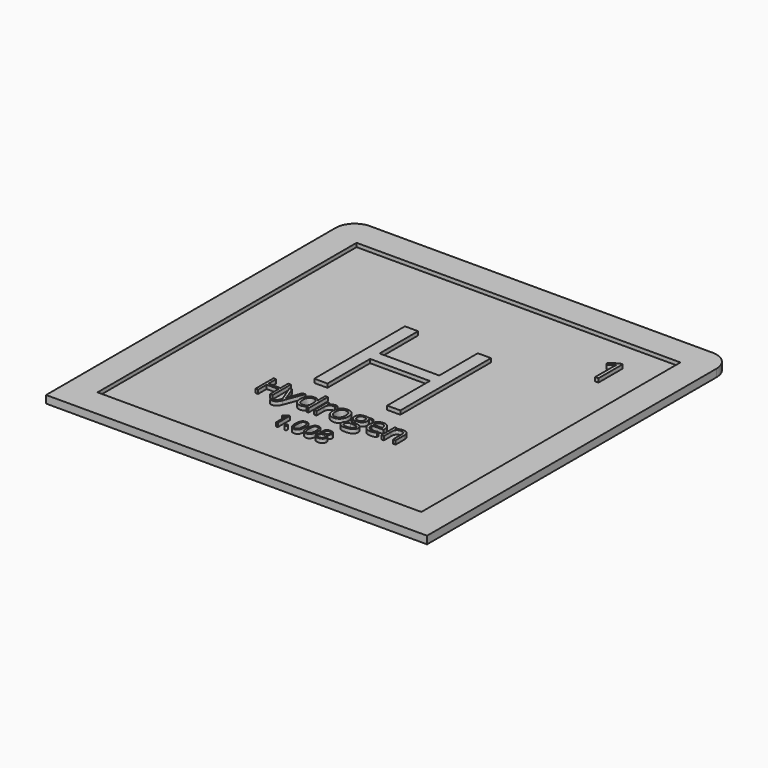
from build123d import *

# Parameters (mm, degrees)
F0_W           = 100
F0_H           = 100
F0_W_2         = 85
F0_H_2         = 85
F0_TEXT_SIZE   = 41.6666666667
F0_TEXT_SIZE_2 = 11.1111111111
F0_TEXT_SIZE_3 = 8.3333333333
F0_TEXT_SIZE_4 = 5.5555555556
F1_DEPTH       = 2
F2_R           = 5
F4_DEPTH       = 1


# Not quite as in the source:
# - Text() gives the source's letters only with a copy of the font that has no kerning and outlines rounded to 1/6400 em; it was checked with that copy


with BuildPart() as f1:
    # F0 (on Top) → F1 (new body)
    with BuildSketch(Plane.XY):
        Rectangle(F0_W, F0_H)
        Rectangle(F0_W_2, F0_H_2, mode=Mode.SUBTRACT)
        with Locations((-15.6875, -10)):
            Text('H', F0_TEXT_SIZE, font='Open Sans', text_align=(TextAlign.LEFT, TextAlign.BOTTOM))
        with Locations((29.9010416667, 26.5)):
            Text('1', F0_TEXT_SIZE_2, font='Open Sans', text_align=(TextAlign.LEFT, TextAlign.BOTTOM))
        with Locations((-19.0579427083, -21)):
            Text('Hydrogen', F0_TEXT_SIZE_3, font='Open Sans', text_align=(TextAlign.LEFT, TextAlign.BOTTOM))
        with Locations((-7.1280381944, -30)):
            Text('1.008', F0_TEXT_SIZE_4, font='Open Sans', text_align=(TextAlign.LEFT, TextAlign.BOTTOM))
    extrude(amount=F1_DEPTH)

    # F2
    f2_edges = [f1.edges().sort_by_distance(p)[0] for p in [
        (50, 50, 1),
        (-50, 50, 1),
    ]]
    fillet(f2_edges, radius=F2_R)

    # F0 (on Top) → F4 (join)
    with BuildSketch(Plane.XY):
        Rectangle(F0_W_2, F0_H_2)
        with BuildLine():
            add(Edge.make_bspline(
                [(-3.4487847222, -29.9934895833), (-3.5394965278, -29.9079861111), (-3.5394965278, -29.7126736111)],
                knots=[0, 0, 0, 1, 1, 1], degree=2))
            add(Edge.make_bspline(
                [(-3.5394965278, -29.7126736111), (-3.5394965278, -29.5303819444), (-3.4565972222, -29.4370659722)],
                knots=[0, 0, 0, 1, 1, 1], degree=2))
            add(Edge.make_bspline(
                [(-3.4565972222, -29.4370659722), (-3.3736979167, -29.34375), (-3.2191840278, -29.34375)],
                knots=[0, 0, 0, 1, 1, 1], degree=2))
            add(Edge.make_bspline(
                [(-3.2191840278, -29.34375), (-3.0620659722, -29.34375), (-2.9739583333, -29.4370659722)],
                knots=[0, 0, 0, 1, 1, 1], degree=2))
            add(Edge.make_bspline(
                [(-2.9739583333, -29.4370659722), (-2.8858506944, -29.5303819444), (-2.8858506944, -29.7126736111)],
                knots=[0, 0, 0, 1, 1, 1], degree=2))
            add(Edge.make_bspline(
                [(-2.8858506944, -29.7126736111), (-2.8858506944, -29.8888888889), (-2.9752604167, -29.9839409722)],
                knots=[0, 0, 0, 1, 1, 1], degree=2))
            add(Edge.make_bspline(
                [(-2.9752604167, -29.9839409722), (-3.0646701389, -30.0789930556), (-3.2191840278, -30.0789930556)],
                knots=[0, 0, 0, 1, 1, 1], degree=2))
            add(Edge.make_bspline(
                [(-3.2191840278, -30.0789930556), (-3.3580729167, -30.0789930556), (-3.4487847222, -29.9934895833)],
                knots=[0, 0, 0, 1, 1, 1], degree=2))
        make_face(mode=Mode.SUBTRACT)
        with BuildLine():
            Line((-5.1888020833, -26.0338541667), (-5.1888020833, -30))
            Line((-5.1888020833, -30), (-5.6280381944, -30))
            Line((-5.6280381944, -30), (-5.6280381944, -27.1736111111))
            add(Edge.make_bspline(
                [(-5.6280381944, -27.1736111111), (-5.6280381944, -26.8203125), (-5.6063368056, -26.5060763889)],
                knots=[0, 0, 0, 1, 1, 1], degree=2))
            add(Edge.make_bspline(
                [(-5.6063368056, -26.5060763889), (-5.6627604167, -26.5633680556), (-5.7335069444, -26.6254340278)],
                knots=[0, 0, 0, 1, 1, 1], degree=2))
            add(Edge.make_bspline(
                [(-5.7335069444, -26.6254340278), (-5.8042534722, -26.6875), (-6.37890625, -27.1545138889)],
                knots=[0, 0, 0, 1, 1, 1], degree=2))
            Line((-6.37890625, -27.1545138889), (-6.6176215278, -26.8454861111))
            Line((-6.6176215278, -26.8454861111), (-5.5681423611, -26.0338541667))
            Line((-5.5681423611, -26.0338541667), (-5.1888020833, -26.0338541667))
        make_face(mode=Mode.SUBTRACT)
        with BuildLine():
            add(Edge.make_bspline(
                [(0.0915798611, -26.4952256944), (0.4266493056, -27.0190972222), (0.4266493056, -28.0112847222)],
                knots=[0, 0, 0, 1, 1, 1], degree=2))
            add(Edge.make_bspline(
                [(0.4266493056, -28.0112847222), (0.4266493056, -29.0399305556), (0.1024305556, -29.5473090278)],
                knots=[0, 0, 0, 1, 1, 1], degree=2))
            add(Edge.make_bspline(
                [(0.1024305556, -29.5473090278), (-0.2217881944, -30.0546875), (-0.8893229167, -30.0546875)],
                knots=[0, 0, 0, 1, 1, 1], degree=2))
            add(Edge.make_bspline(
                [(-0.8893229167, -30.0546875), (-1.5290798611, -30.0546875), (-1.8628472222, -29.53515625)],
                knots=[0, 0, 0, 1, 1, 1], degree=2))
            add(Edge.make_bspline(
                [(-1.8628472222, -29.53515625), (-2.1966145833, -29.015625), (-2.1966145833, -28.0112847222)],
                knots=[0, 0, 0, 1, 1, 1], degree=2))
            add(Edge.make_bspline(
                [(-2.1966145833, -28.0112847222), (-2.1966145833, -26.9756944444), (-1.8736979167, -26.4735243056)],
                knots=[0, 0, 0, 1, 1, 1], degree=2))
            add(Edge.make_bspline(
                [(-1.8736979167, -26.4735243056), (-1.55078125, -25.9713541667), (-0.8893229167, -25.9713541667)],
                knots=[0, 0, 0, 1, 1, 1], degree=2))
            add(Edge.make_bspline(
                [(-0.8893229167, -25.9713541667), (-0.2434895833, -25.9713541667), (0.0915798611, -26.4952256944)],
                knots=[0, 0, 0, 1, 1, 1], degree=2))
        make_face(mode=Mode.SUBTRACT)
        Polygon((-13.7233072917, -15.05078125), (-13.7233072917, -21), (-14.4147135417, -21), (-14.4147135417, -18.2005208333), (-17.548828125, -18.2005208333), (-17.548828125, -21), (-18.240234375, -21), (-18.240234375, -15.05078125), (-17.548828125, -15.05078125), (-17.548828125, -17.58203125), (-14.4147135417, -17.58203125), (-14.4147135417, -15.05078125), align=None, mode=Mode.SUBTRACT)
        with BuildLine():
            Line((-11.1022135417, -21.0247395833), (-12.9016927083, -16.5403645833))
            Line((-12.9016927083, -16.5403645833), (-12.1764322917, -16.5403645833))
            Line((-12.1764322917, -16.5403645833), (-11.1998697917, -19.0833333333))
            add(Edge.make_bspline(
                [(-11.1998697917, -19.0833333333), (-10.8795572917, -19.9544270833), (-10.8014322917, -20.3411458333)],
                knots=[0, 0, 0, 1, 1, 1], degree=2))
            Line((-10.8014322917, -20.3411458333), (-10.7688802083, -20.3411458333))
            add(Edge.make_bspline(
                [(-10.7688802083, -20.3411458333), (-10.716796875, -20.1328125), (-10.5475260417, -19.6302083333)],
                knots=[0, 0, 0, 1, 1, 1], degree=2))
            add(Edge.make_bspline(
                [(-10.5475260417, -19.6302083333), (-10.3782552083, -19.1276041667), (-9.4420572917, -16.5403645833)],
                knots=[0, 0, 0, 1, 1, 1], degree=2))
            Line((-9.4420572917, -16.5403645833), (-8.7180989583, -16.5403645833))
            Line((-8.7180989583, -16.5403645833), (-10.634765625, -21.6184895833))
            add(Edge.make_bspline(
                [(-10.634765625, -21.6184895833), (-10.919921875, -22.37109375), (-11.3001302083, -22.6868489583)],
                knots=[0, 0, 0, 1, 1, 1], degree=2))
            add(Edge.make_bspline(
                [(-11.3001302083, -22.6868489583), (-11.6803385417, -23.0026041667), (-12.2337239583, -23.0026041667)],
                knots=[0, 0, 0, 1, 1, 1], degree=2))
            add(Edge.make_bspline(
                [(-12.2337239583, -23.0026041667), (-12.5436197917, -23.0026041667), (-12.8444010417, -22.9322916667)],
                knots=[0, 0, 0, 1, 1, 1], degree=2))
            Line((-12.8444010417, -22.9322916667), (-12.8444010417, -22.3919270833))
            add(Edge.make_bspline(
                [(-12.8444010417, -22.3919270833), (-12.6204427083, -22.4401041667), (-12.3444010417, -22.4401041667)],
                knots=[0, 0, 0, 1, 1, 1], degree=2))
            add(Edge.make_bspline(
                [(-12.3444010417, -22.4401041667), (-11.6477864583, -22.4401041667), (-11.3509114583, -21.6588541667)],
                knots=[0, 0, 0, 1, 1, 1], degree=2))
            Line((-11.3509114583, -21.6588541667), (-11.1022135417, -21.0247395833))
        make_face(mode=Mode.SUBTRACT)
        with BuildLine():
            Line((-4.869140625, -21), (-4.958984375, -20.40234375))
            Line((-4.958984375, -20.40234375), (-4.9954427083, -20.40234375))
            add(Edge.make_bspline(
                [(-4.9954427083, -20.40234375), (-5.462890625, -21.08203125), (-6.3951822917, -21.08203125)],
                knots=[0, 0, 0, 1, 1, 1], degree=2))
            add(Edge.make_bspline(
                [(-6.3951822917, -21.08203125), (-7.2701822917, -21.08203125), (-7.7565104167, -20.4837239583)],
                knots=[0, 0, 0, 1, 1, 1], degree=2))
            add(Edge.make_bspline(
                [(-7.7565104167, -20.4837239583), (-8.2428385417, -19.8854166667), (-8.2428385417, -18.7825520833)],
                knots=[0, 0, 0, 1, 1, 1], degree=2))
            add(Edge.make_bspline(
                [(-8.2428385417, -18.7825520833), (-8.2428385417, -17.6796875), (-7.7545572917, -17.0690104167)],
                knots=[0, 0, 0, 1, 1, 1], degree=2))
            add(Edge.make_bspline(
                [(-7.7545572917, -17.0690104167), (-7.2662760417, -16.4583333333), (-6.3951822917, -16.4583333333)],
                knots=[0, 0, 0, 1, 1, 1], degree=2))
            add(Edge.make_bspline(
                [(-6.3951822917, -16.4583333333), (-5.4876302083, -16.4583333333), (-5.0032552083, -17.1184895833)],
                knots=[0, 0, 0, 1, 1, 1], degree=2))
            Line((-5.0032552083, -17.1184895833), (-4.9498697917, -17.1184895833))
            Line((-4.9498697917, -17.1184895833), (-4.978515625, -16.796875))
            Line((-4.978515625, -16.796875), (-4.9954427083, -16.4830729167))
            Line((-4.9954427083, -16.4830729167), (-4.9954427083, -14.66796875))
            Line((-4.9954427083, -14.66796875), (-4.3196614583, -14.66796875))
            Line((-4.3196614583, -14.66796875), (-4.3196614583, -21))
            Line((-4.3196614583, -21), (-4.869140625, -21))
        make_face(mode=Mode.SUBTRACT)
        with BuildLine():
            add(Edge.make_bspline(
                [(-1.6217447917, -16.6946614583), (-1.271484375, -16.4583333333), (-0.8522135417, -16.4583333333)],
                knots=[0, 0, 0, 1, 1, 1], degree=2))
            add(Edge.make_bspline(
                [(-0.8522135417, -16.4583333333), (-0.5553385417, -16.4583333333), (-0.3196614583, -16.5078125)],
                knots=[0, 0, 0, 1, 1, 1], degree=2))
            Line((-0.3196614583, -16.5078125), (-0.4134114583, -17.1341145833))
            add(Edge.make_bspline(
                [(-0.4134114583, -17.1341145833), (-0.689453125, -17.0729166667), (-0.9016927083, -17.0729166667)],
                knots=[0, 0, 0, 1, 1, 1], degree=2))
            add(Edge.make_bspline(
                [(-0.9016927083, -17.0729166667), (-1.443359375, -17.0729166667), (-1.8274739583, -17.5123697917)],
                knots=[0, 0, 0, 1, 1, 1], degree=2))
            add(Edge.make_bspline(
                [(-1.8274739583, -17.5123697917), (-2.2115885417, -17.9518229167), (-2.2115885417, -18.6067708333)],
                knots=[0, 0, 0, 1, 1, 1], degree=2))
            Line((-2.2115885417, -18.6067708333), (-2.2115885417, -21))
            Line((-2.2115885417, -21), (-2.8873697917, -21))
            Line((-2.8873697917, -21), (-2.8873697917, -16.5403645833))
            Line((-2.8873697917, -16.5403645833), (-2.330078125, -16.5403645833))
            Line((-2.330078125, -16.5403645833), (-2.251953125, -17.3658854167))
            Line((-2.251953125, -17.3658854167), (-2.2194010417, -17.3658854167))
            add(Edge.make_bspline(
                [(-2.2194010417, -17.3658854167), (-1.9720052083, -16.9309895833), (-1.6217447917, -16.6946614583)],
                knots=[0, 0, 0, 1, 1, 1], degree=2))
        make_face(mode=Mode.SUBTRACT)
        with BuildLine():
            add(Edge.make_bspline(
                [(3.2677951389, -26.4952256944), (3.6028645833, -27.0190972222), (3.6028645833, -28.0112847222)],
                knots=[0, 0, 0, 1, 1, 1], degree=2))
            add(Edge.make_bspline(
                [(3.6028645833, -28.0112847222), (3.6028645833, -29.0399305556), (3.2786458333, -29.5473090278)],
                knots=[0, 0, 0, 1, 1, 1], degree=2))
            add(Edge.make_bspline(
                [(3.2786458333, -29.5473090278), (2.9544270833, -30.0546875), (2.2868923611, -30.0546875)],
                knots=[0, 0, 0, 1, 1, 1], degree=2))
            add(Edge.make_bspline(
                [(2.2868923611, -30.0546875), (1.6471354167, -30.0546875), (1.3133680556, -29.53515625)],
                knots=[0, 0, 0, 1, 1, 1], degree=2))
            add(Edge.make_bspline(
                [(1.3133680556, -29.53515625), (0.9796006944, -29.015625), (0.9796006944, -28.0112847222)],
                knots=[0, 0, 0, 1, 1, 1], degree=2))
            add(Edge.make_bspline(
                [(0.9796006944, -28.0112847222), (0.9796006944, -26.9756944444), (1.3025173611, -26.4735243056)],
                knots=[0, 0, 0, 1, 1, 1], degree=2))
            add(Edge.make_bspline(
                [(1.3025173611, -26.4735243056), (1.6254340278, -25.9713541667), (2.2868923611, -25.9713541667)],
                knots=[0, 0, 0, 1, 1, 1], degree=2))
            add(Edge.make_bspline(
                [(2.2868923611, -25.9713541667), (2.9327256944, -25.9713541667), (3.2677951389, -26.4952256944)],
                knots=[0, 0, 0, 1, 1, 1], degree=2))
        make_face(mode=Mode.SUBTRACT)
        with BuildLine():
            add(Edge.make_bspline(
                [(4.6098090278, -26.2335069444), (4.9283854167, -25.9774305556), (5.4631076389, -25.9774305556)],
                knots=[0, 0, 0, 1, 1, 1], degree=2))
            add(Edge.make_bspline(
                [(5.4631076389, -25.9774305556), (6.0056423611, -25.9774305556), (6.3229166667, -26.2296006944)],
                knots=[0, 0, 0, 1, 1, 1], degree=2))
            add(Edge.make_bspline(
                [(6.3229166667, -26.2296006944), (6.6401909722, -26.4817708333), (6.6401909722, -26.9262152778)],
                knots=[0, 0, 0, 1, 1, 1], degree=2))
            add(Edge.make_bspline(
                [(6.6401909722, -26.9262152778), (6.6401909722, -27.2196180556), (6.4587673611, -27.4609375)],
                knots=[0, 0, 0, 1, 1, 1], degree=2))
            add(Edge.make_bspline(
                [(6.4587673611, -27.4609375), (6.27734375, -27.7022569444), (5.8780381944, -27.9001736111)],
                knots=[0, 0, 0, 1, 1, 1], degree=2))
            add(Edge.make_bspline(
                [(5.8780381944, -27.9001736111), (6.3606770833, -28.1310763889), (6.5642361111, -28.3845486111)],
                knots=[0, 0, 0, 1, 1, 1], degree=2))
            add(Edge.make_bspline(
                [(6.5642361111, -28.3845486111), (6.7677951389, -28.6380208333), (6.7677951389, -28.9722222222)],
                knots=[0, 0, 0, 1, 1, 1], degree=2))
            add(Edge.make_bspline(
                [(6.7677951389, -28.9722222222), (6.7677951389, -29.4652777778), (6.4231770833, -29.7599826389)],
                knots=[0, 0, 0, 1, 1, 1], degree=2))
            add(Edge.make_bspline(
                [(6.4231770833, -29.7599826389), (6.0785590278, -30.0546875), (5.4796006944, -30.0546875)],
                knots=[0, 0, 0, 1, 1, 1], degree=2))
            add(Edge.make_bspline(
                [(5.4796006944, -30.0546875), (4.8450520833, -30.0546875), (4.5030381944, -29.7764756944)],
                knots=[0, 0, 0, 1, 1, 1], degree=2))
            add(Edge.make_bspline(
                [(4.5030381944, -29.7764756944), (4.1610243056, -29.4982638889), (4.1610243056, -28.9878472222)],
                knots=[0, 0, 0, 1, 1, 1], degree=2))
            add(Edge.make_bspline(
                [(4.1610243056, -28.9878472222), (4.1610243056, -28.3072916667), (4.9908854167, -27.9270833333)],
                knots=[0, 0, 0, 1, 1, 1], degree=2))
            add(Edge.make_bspline(
                [(4.9908854167, -27.9270833333), (4.6167534722, -27.7161458333), (4.4539930556, -27.4704861111)],
                knots=[0, 0, 0, 1, 1, 1], degree=2))
            add(Edge.make_bspline(
                [(4.4539930556, -27.4704861111), (4.2912326389, -27.2248263889), (4.2912326389, -26.9210069444)],
                knots=[0, 0, 0, 1, 1, 1], degree=2))
            add(Edge.make_bspline(
                [(4.2912326389, -26.9210069444), (4.2912326389, -26.4895833333), (4.6098090278, -26.2335069444)],
                knots=[0, 0, 0, 1, 1, 1], degree=2))
        make_face(mode=Mode.SUBTRACT)
        with BuildLine():
            add(Edge.make_bspline(
                [(3.8125, -17.0813802083), (4.3639322917, -17.7044270833), (4.3639322917, -18.765625)],
                knots=[0, 0, 0, 1, 1, 1], degree=2))
            add(Edge.make_bspline(
                [(4.3639322917, -18.765625), (4.3639322917, -19.8567708333), (3.8151041667, -20.4694010417)],
                knots=[0, 0, 0, 1, 1, 1], degree=2))
            add(Edge.make_bspline(
                [(3.8151041667, -20.4694010417), (3.2662760417, -21.08203125), (2.2975260417, -21.08203125)],
                knots=[0, 0, 0, 1, 1, 1], degree=2))
            add(Edge.make_bspline(
                [(2.2975260417, -21.08203125), (1.6985677083, -21.08203125), (1.2350260417, -20.80078125)],
                knots=[0, 0, 0, 1, 1, 1], degree=2))
            add(Edge.make_bspline(
                [(1.2350260417, -20.80078125), (0.771484375, -20.51953125), (0.5188802083, -19.9947916667)],
                knots=[0, 0, 0, 1, 1, 1], degree=2))
            add(Edge.make_bspline(
                [(0.5188802083, -19.9947916667), (0.2662760417, -19.4700520833), (0.2662760417, -18.765625)],
                knots=[0, 0, 0, 1, 1, 1], degree=2))
            add(Edge.make_bspline(
                [(0.2662760417, -18.765625), (0.2662760417, -17.67578125), (0.8118489583, -17.0670572917)],
                knots=[0, 0, 0, 1, 1, 1], degree=2))
            add(Edge.make_bspline(
                [(0.8118489583, -17.0670572917), (1.357421875, -16.4583333333), (2.326171875, -16.4583333333)],
                knots=[0, 0, 0, 1, 1, 1], degree=2))
            add(Edge.make_bspline(
                [(2.326171875, -16.4583333333), (3.2610677083, -16.4583333333), (3.8125, -17.0813802083)],
                knots=[0, 0, 0, 1, 1, 1], degree=2))
        make_face(mode=Mode.SUBTRACT)
        with BuildLine():
            Line((7.6569010417, -16.5403645833), (9.1985677083, -16.5403645833))
            Line((9.1985677083, -16.5403645833), (9.1985677083, -16.9674479167))
            Line((9.1985677083, -16.9674479167), (8.373046875, -17.0651041667))
            add(Edge.make_bspline(
                [(8.373046875, -17.0651041667), (8.486328125, -17.20703125), (8.576171875, -17.4375)],
                knots=[0, 0, 0, 1, 1, 1], degree=2))
            add(Edge.make_bspline(
                [(8.576171875, -17.4375), (8.666015625, -17.66796875), (8.666015625, -17.9557291667)],
                knots=[0, 0, 0, 1, 1, 1], degree=2))
            add(Edge.make_bspline(
                [(8.666015625, -17.9557291667), (8.666015625, -18.6119791667), (8.2180989583, -19.0026041667)],
                knots=[0, 0, 0, 1, 1, 1], degree=2))
            add(Edge.make_bspline(
                [(8.2180989583, -19.0026041667), (7.7701822917, -19.3932291667), (6.9889322917, -19.3932291667)],
                knots=[0, 0, 0, 1, 1, 1], degree=2))
            add(Edge.make_bspline(
                [(6.9889322917, -19.3932291667), (6.7897135417, -19.3932291667), (6.615234375, -19.3606770833)],
                knots=[0, 0, 0, 1, 1, 1], degree=2))
            add(Edge.make_bspline(
                [(6.615234375, -19.3606770833), (6.1842447917, -19.5885416667), (6.1842447917, -19.93359375)],
                knots=[0, 0, 0, 1, 1, 1], degree=2))
            add(Edge.make_bspline(
                [(6.1842447917, -19.93359375), (6.1842447917, -20.1171875), (6.3346354167, -20.2044270833)],
                knots=[0, 0, 0, 1, 1, 1], degree=2))
            add(Edge.make_bspline(
                [(6.3346354167, -20.2044270833), (6.4850260417, -20.2916666667), (6.8509114583, -20.2916666667)],
                knots=[0, 0, 0, 1, 1, 1], degree=2))
            Line((6.8509114583, -20.2916666667), (7.6399739583, -20.2916666667))
            add(Edge.make_bspline(
                [(7.6399739583, -20.2916666667), (8.365234375, -20.2916666667), (8.7532552083, -20.5970052083)],
                knots=[0, 0, 0, 1, 1, 1], degree=2))
            add(Edge.make_bspline(
                [(8.7532552083, -20.5970052083), (9.1412760417, -20.90234375), (9.1412760417, -21.484375)],
                knots=[0, 0, 0, 1, 1, 1], degree=2))
            add(Edge.make_bspline(
                [(9.1412760417, -21.484375), (9.1412760417, -22.2252604167), (8.5475260417, -22.6139322917)],
                knots=[0, 0, 0, 1, 1, 1], degree=2))
            add(Edge.make_bspline(
                [(8.5475260417, -22.6139322917), (7.9537760417, -23.0026041667), (6.814453125, -23.0026041667)],
                knots=[0, 0, 0, 1, 1, 1], degree=2))
            add(Edge.make_bspline(
                [(6.814453125, -23.0026041667), (5.939453125, -23.0026041667), (5.4654947917, -22.6770833333)],
                knots=[0, 0, 0, 1, 1, 1], degree=2))
            add(Edge.make_bspline(
                [(5.4654947917, -22.6770833333), (4.9915364583, -22.3515625), (4.9915364583, -21.7565104167)],
                knots=[0, 0, 0, 1, 1, 1], degree=2))
            add(Edge.make_bspline(
                [(4.9915364583, -21.7565104167), (4.9915364583, -21.3502604167), (5.251953125, -21.052734375)],
                knots=[0, 0, 0, 1, 1, 1], degree=2))
            add(Edge.make_bspline(
                [(5.251953125, -21.052734375), (5.5123697917, -20.7552083333), (5.9837239583, -20.6497395833)],
                knots=[0, 0, 0, 1, 1, 1], degree=2))
            add(Edge.make_bspline(
                [(5.9837239583, -20.6497395833), (5.8131510417, -20.5729166667), (5.697265625, -20.41015625)],
                knots=[0, 0, 0, 1, 1, 1], degree=2))
            add(Edge.make_bspline(
                [(5.697265625, -20.41015625), (5.5813802083, -20.2473958333), (5.5813802083, -20.03125)],
                knots=[0, 0, 0, 1, 1, 1], degree=2))
            add(Edge.make_bspline(
                [(5.5813802083, -20.03125), (5.5813802083, -19.7877604167), (5.7115885417, -19.6041666667)],
                knots=[0, 0, 0, 1, 1, 1], degree=2))
            add(Edge.make_bspline(
                [(5.7115885417, -19.6041666667), (5.841796875, -19.4205729167), (6.123046875, -19.25)],
                knots=[0, 0, 0, 1, 1, 1], degree=2))
            add(Edge.make_bspline(
                [(6.123046875, -19.25), (5.7766927083, -19.1080729167), (5.5592447917, -18.7662760417)],
                knots=[0, 0, 0, 1, 1, 1], degree=2))
            add(Edge.make_bspline(
                [(5.5592447917, -18.7662760417), (5.341796875, -18.4244791667), (5.341796875, -17.984375)],
                knots=[0, 0, 0, 1, 1, 1], degree=2))
            add(Edge.make_bspline(
                [(5.341796875, -17.984375), (5.341796875, -17.2526041667), (5.78125, -16.85546875)],
                knots=[0, 0, 0, 1, 1, 1], degree=2))
            add(Edge.make_bspline(
                [(5.78125, -16.85546875), (6.220703125, -16.4583333333), (7.025390625, -16.4583333333)],
                knots=[0, 0, 0, 1, 1, 1], degree=2))
            add(Edge.make_bspline(
                [(7.025390625, -16.4583333333), (7.3756510417, -16.4583333333), (7.6569010417, -16.5403645833)],
                knots=[0, 0, 0, 1, 1, 1], degree=2))
        make_face(mode=Mode.SUBTRACT)
        with BuildLine():
            add(Edge.make_bspline(
                [(12.7688802083, -21.0143229167), (12.4498697917, -21.08203125), (11.998046875, -21.08203125)],
                knots=[0, 0, 0, 1, 1, 1], degree=2))
            add(Edge.make_bspline(
                [(11.998046875, -21.08203125), (11.009765625, -21.08203125), (10.4375, -20.4791666667)],
                knots=[0, 0, 0, 1, 1, 1], degree=2))
            add(Edge.make_bspline(
                [(10.4375, -20.4791666667), (9.865234375, -19.8763020833), (9.865234375, -18.8072916667)],
                knots=[0, 0, 0, 1, 1, 1], degree=2))
            add(Edge.make_bspline(
                [(9.865234375, -18.8072916667), (9.865234375, -17.7278645833), (10.396484375, -17.0930989583)],
                knots=[0, 0, 0, 1, 1, 1], degree=2))
            add(Edge.make_bspline(
                [(10.396484375, -17.0930989583), (10.927734375, -16.4583333333), (11.8235677083, -16.4583333333)],
                knots=[0, 0, 0, 1, 1, 1], degree=2))
            add(Edge.make_bspline(
                [(11.8235677083, -16.4583333333), (12.6608072917, -16.4583333333), (13.1490885417, -17.009765625)],
                knots=[0, 0, 0, 1, 1, 1], degree=2))
            add(Edge.make_bspline(
                [(13.1490885417, -17.009765625), (13.6373697917, -17.5611979167), (13.6373697917, -18.46484375)],
                knots=[0, 0, 0, 1, 1, 1], degree=2))
            Line((13.6373697917, -18.46484375), (13.6373697917, -18.8919270833))
            Line((13.6373697917, -18.8919270833), (10.5657552083, -18.8919270833))
            add(Edge.make_bspline(
                [(10.5657552083, -18.8919270833), (10.5865885417, -19.6770833333), (10.962890625, -20.083984375)],
                knots=[0, 0, 0, 1, 1, 1], degree=2))
            add(Edge.make_bspline(
                [(10.962890625, -20.083984375), (11.3391927083, -20.4908854167), (12.0227864583, -20.4908854167)],
                knots=[0, 0, 0, 1, 1, 1], degree=2))
            add(Edge.make_bspline(
                [(12.0227864583, -20.4908854167), (12.7428385417, -20.4908854167), (13.4459635417, -20.1901041667)],
                knots=[0, 0, 0, 1, 1, 1], degree=2))
            Line((13.4459635417, -20.1901041667), (13.4459635417, -20.79296875))
            add(Edge.make_bspline(
                [(13.4459635417, -20.79296875), (13.087890625, -20.9466145833), (12.7688802083, -21.0143229167)],
                knots=[0, 0, 0, 1, 1, 1], degree=2))
        make_face(mode=Mode.SUBTRACT)
        with BuildLine():
            Line((18.517578125, -21), (17.841796875, -21))
            Line((17.841796875, -21), (17.841796875, -18.1145833333))
            add(Edge.make_bspline(
                [(17.841796875, -18.1145833333), (17.841796875, -17.5703125), (17.59375, -17.3014322917)],
                knots=[0, 0, 0, 1, 1, 1], degree=2))
            add(Edge.make_bspline(
                [(17.59375, -17.3014322917), (17.345703125, -17.0325520833), (16.8157552083, -17.0325520833)],
                knots=[0, 0, 0, 1, 1, 1], degree=2))
            add(Edge.make_bspline(
                [(16.8157552083, -17.0325520833), (16.1165364583, -17.0325520833), (15.791015625, -17.4108072917)],
                knots=[0, 0, 0, 1, 1, 1], degree=2))
            add(Edge.make_bspline(
                [(15.791015625, -17.4108072917), (15.4654947917, -17.7890625), (15.4654947917, -18.66015625)],
                knots=[0, 0, 0, 1, 1, 1], degree=2))
            Line((15.4654947917, -18.66015625), (15.4654947917, -21))
            Line((15.4654947917, -21), (14.7897135417, -21))
            Line((14.7897135417, -21), (14.7897135417, -16.5403645833))
            Line((14.7897135417, -16.5403645833), (15.3391927083, -16.5403645833))
            Line((15.3391927083, -16.5403645833), (15.4485677083, -17.1510416667))
            Line((15.4485677083, -17.1510416667), (15.4811197917, -17.1510416667))
            add(Edge.make_bspline(
                [(15.4811197917, -17.1510416667), (15.689453125, -16.8216145833), (16.0638020833, -16.6399739583)],
                knots=[0, 0, 0, 1, 1, 1], degree=2))
            add(Edge.make_bspline(
                [(16.0638020833, -16.6399739583), (16.4381510417, -16.4583333333), (16.8977864583, -16.4583333333)],
                knots=[0, 0, 0, 1, 1, 1], degree=2))
            add(Edge.make_bspline(
                [(16.8977864583, -16.4583333333), (17.7037760417, -16.4583333333), (18.1106770833, -16.8470052083)],
                knots=[0, 0, 0, 1, 1, 1], degree=2))
            add(Edge.make_bspline(
                [(18.1106770833, -16.8470052083), (18.517578125, -17.2356770833), (18.517578125, -18.0911458333)],
                knots=[0, 0, 0, 1, 1, 1], degree=2))
            Line((18.517578125, -18.0911458333), (18.517578125, -21))
        make_face(mode=Mode.SUBTRACT)
        Polygon((10.9856770833, 19.74609375), (10.9856770833, -10), (7.5286458333, -10), (7.5286458333, 3.9973958333), (-8.1419270833, 3.9973958333), (-8.1419270833, -10), (-11.5989583333, -10), (-11.5989583333, 19.74609375), (-8.1419270833, 19.74609375), (-8.1419270833, 7.08984375), (7.5286458333, 7.08984375), (7.5286458333, 19.74609375), align=None, mode=Mode.SUBTRACT)
        with BuildLine():
            Line((33.7795138889, 34.4322916667), (33.7795138889, 26.5))
            Line((33.7795138889, 26.5), (32.9010416667, 26.5))
            Line((32.9010416667, 26.5), (32.9010416667, 32.1527777778))
            add(Edge.make_bspline(
                [(32.9010416667, 32.1527777778), (32.9010416667, 32.859375), (32.9444444444, 33.4878472222)],
                knots=[0, 0, 0, 1, 1, 1], degree=2))
            add(Edge.make_bspline(
                [(32.9444444444, 33.4878472222), (32.8315972222, 33.3732638889), (32.6901041667, 33.2491319444)],
                knots=[0, 0, 0, 1, 1, 1], degree=2))
            add(Edge.make_bspline(
                [(32.6901041667, 33.2491319444), (32.5486111111, 33.125), (31.3993055556, 32.1909722222)],
                knots=[0, 0, 0, 1, 1, 1], degree=2))
            Line((31.3993055556, 32.1909722222), (30.921875, 32.8090277778))
            Line((30.921875, 32.8090277778), (33.0208333333, 34.4322916667))
            Line((33.0208333333, 34.4322916667), (33.7795138889, 34.4322916667))
        make_face(mode=Mode.SUBTRACT)
    extrude(amount=F4_DEPTH)


solid = f1.part
